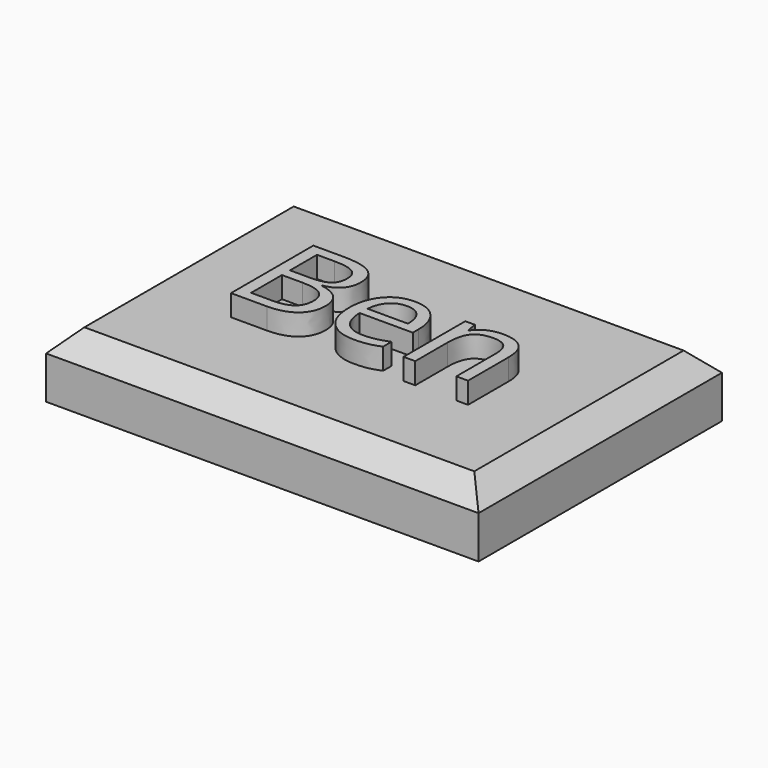
from build123d import *

# Parameters (mm, degrees)
F0_W         = 101.6
F0_H         = 71.4644104478
F1_DEPTH     = 15
F2_TEXT_SIZE = 33.8684004318
F3_DEPTH     = 20
F4_SIZE      = 5


# Not quite as in the source:
# - a feature names something its author has since deleted; it is built from what else it names
# - Text() gives the source's letters only with a copy of the font that has no kerning and outlines rounded to 1/6400 em; it was checked with that copy


with BuildPart() as f1:
    # F0 (on Top) → F1 (new body)
    with BuildSketch(Plane.XY):
        Rectangle(F0_W, F0_H)
    extrude(amount=F1_DEPTH)

    # F2 (on Top) → F3 (join)
    with BuildSketch(Plane.XY):
        with Locations((-30.6032749526, -10.8311213553)):
            Text('Ben', F2_TEXT_SIZE, font='Open Sans', text_align=(TextAlign.LEFT, TextAlign.BOTTOM))
    extrude(amount=F3_DEPTH)

    # F4
    f4_edges = [f1.edges().sort_by_distance(p)[0] for p in [
        (0, 35.732205, 15),
        (50.8, 0, 15),
        (0, -35.732205, 15),
        (-50.8, 0, 15),
    ]]
    chamfer(f4_edges, length=F4_SIZE)


solid = f1.part
